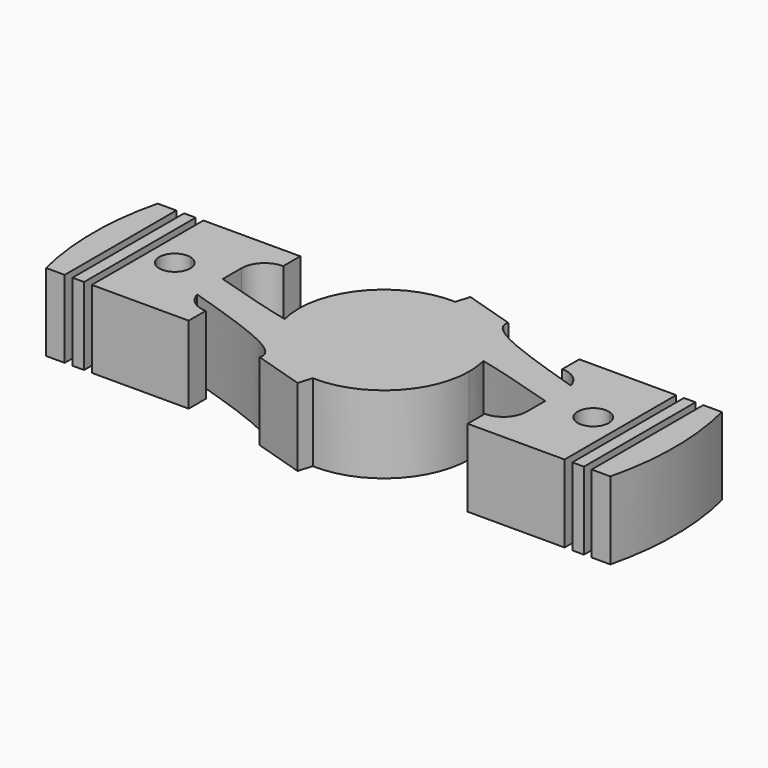
from build123d import *

# Parameters (mm, degrees)
F0_DEPTH = 25.4
F1_W     = 3.81
F1_H     = 45.72


with BuildPart() as f0:
    # F1 (on Top) → F0 (new body)
    with BuildSketch(Plane.XY):
        with BuildLine():
            Line((77.47, 22.86), (45.72, 22.86))
            Line((45.72, 22.86), (45.72, 15.875))
            ThreePointArc((45.72, 15.875), (50.3897919484, 14.2764153784), (53.1002511947, 10.1513892806))
            add(Edge.make_bspline(
                [(53.1002511947, 10.1513892806), (58.1589510072, 8.551724236), (63.812727866, 6.7977717351), (70.0851851843, 4.8518880408)],
                knots=[46.5844881463, 46.5844881463, 46.5844881463, 46.5844881463, 55.8862582945, 55.8862582945, 55.8862582945, 55.8862582945], degree=3))
            ThreePointArc((70.0851851843, 4.8518880408), (72.6697885481, 3.0133087515), (73.66, 0))
            ThreePointArc((73.66, 0), (71.5933087511, -4.0897885484), (67.0748148148, -4.8518880406))
            add(Edge.make_bspline(
                [(53.34, -0.6059576), (57.5451254916, -1.8955240295), (62.1166858374, -3.3137440808), (67.0748148148, -4.8518880406)],
                knots=[48.5335775556, 48.5335775556, 48.5335775556, 48.5335775556, 55.8862582953, 55.8862582953, 55.8862582953, 55.8862582953], degree=3))
            Line((53.34, -0.6059576), (53.34, -8.255))
            ThreePointArc((53.34, -8.255), (51.1081536726, -13.6431536726), (45.72, -15.875))
            Line((45.72, -15.875), (45.72, -22.86))
            Line((45.72, -22.86), (77.47, -22.86))
            Line((77.47, -22.86), (77.47, 22.86))
        make_face()
        with BuildLine():
            add(Edge.make_bspline(
                [(53.1002511947, 10.1513892806), (58.1589510072, 8.551724236), (63.812727866, 6.7977717351), (70.0851851843, 4.8518880408)],
                knots=[46.5844881463, 46.5844881463, 46.5844881463, 46.5844881463, 55.8862582945, 55.8862582945, 55.8862582945, 55.8862582945], degree=3))
            ThreePointArc((53.1002511947, 10.1513892806), (53.2798251998, 9.210742093), (53.34, 8.255))
            Line((53.34, 8.255), (53.34, -0.6059576))
            add(Edge.make_bspline(
                [(53.34, -0.6059576), (57.5451254916, -1.8955240295), (62.1166858374, -3.3137440808), (67.0748148148, -4.8518880406)],
                knots=[48.5335775556, 48.5335775556, 48.5335775556, 48.5335775556, 55.8862582953, 55.8862582953, 55.8862582953, 55.8862582953], degree=3))
            ThreePointArc((67.0748148148, -4.8518880406), (63.7281119593, 1.5051851848), (70.0851851843, 4.8518880408))
        make_face()
        with BuildLine():
            ThreePointArc((53.34, 8.255), (53.2798251998, 9.210742093), (53.1002511947, 10.1513892806))
            add(Edge.make_bspline(
                [(18.9075672089, 27.3046224959), (17.3563376005, 22.3043125946), (27.7656172811, 18.1627221903), (53.1002511947, 10.1513892806)],
                knots=[0, 0, 0, 0, 46.5844881463, 46.5844881463, 46.5844881463, 46.5844881463], degree=3))
            Line((18.9075672089, 27.3046224959), (2.4020174164, 32.4250846362))
            Line((2.4020174164, 32.4250846362), (1.0050151405, 27.9219187121))
            ThreePointArc((1.0050151405, 27.9219187121), (17.5750428532, 21.7200706423), (27.0976887869, 6.8087342735))
            add(Edge.make_bspline(
                [(27.0976887869, 6.8087342735), (33.4853412167, 5.3665593675), (42.104777648, 2.8394961928), (53.34, -0.6059576)],
                knots=[28.888740996, 28.888740996, 28.888740996, 28.888740996, 48.5335775556, 48.5335775556, 48.5335775556, 48.5335775556], degree=3))
            Line((53.34, -0.6059576), (53.34, 8.255))
        make_face()
        with BuildLine():
            ThreePointArc((27.94, 0), (27.7286226191, 3.4303188841), (27.0976887869, 6.8087342735))
            ThreePointArc((27.0976887869, 6.8087342735), (17.5750428532, 21.7200706423), (1.0050151405, 27.9219187121))
            ThreePointArc((1.0050151405, 27.9219187121), (-21.7200706423, 17.5750428532), (-27.0976887869, -6.8087342735))
            ThreePointArc((-27.0976887869, -6.8087342735), (-17.5750428532, -21.7200706423), (-1.0050151405, -27.9219187121))
            ThreePointArc((-1.0050151405, -27.9219187121), (19.3979828458, -20.108750869), (27.94, 0))
        make_face()
        with BuildLine():
            ThreePointArc((-1.0050151405, -27.9219187121), (-17.5750428532, -21.7200706423), (-27.0976887869, -6.8087342735))
            add(Edge.make_bspline(
                [(-27.0976887869, -6.8087342735), (-33.4853412167, -5.3665593675), (-42.104777648, -2.8394961928), (-53.34, 0.6059576)],
                knots=[28.888740996, 28.888740996, 28.888740996, 28.888740996, 48.5335775556, 48.5335775556, 48.5335775556, 48.5335775556], degree=3))
            Line((-53.34, 0.6059576), (-53.34, -8.255))
            ThreePointArc((-53.34, -8.255), (-53.2798251998, -9.210742093), (-53.1002511947, -10.1513892806))
            add(Edge.make_bspline(
                [(-18.9075672089, -27.3046224959), (-17.3563376005, -22.3043125946), (-27.7656172811, -18.1627221903), (-53.1002511947, -10.1513892806)],
                knots=[0, 0, 0, 0, 46.5844881463, 46.5844881463, 46.5844881463, 46.5844881463], degree=3))
            Line((-18.9075672089, -27.3046224959), (-2.4020174164, -32.4250846362))
            Line((-2.4020174164, -32.4250846362), (-1.0050151405, -27.9219187121))
        make_face()
        with BuildLine():
            add(Edge.make_bspline(
                [(-53.34, 0.6059576), (-57.5451254916, 1.8955240295), (-62.1166858374, 3.3137440808), (-67.0748148148, 4.8518880406)],
                knots=[48.5335775556, 48.5335775556, 48.5335775556, 48.5335775556, 55.8862582953, 55.8862582953, 55.8862582953, 55.8862582953], degree=3))
            Line((-53.34, 0.6059576), (-53.34, 8.255))
            ThreePointArc((-53.34, 8.255), (-51.1081536726, 13.6431536726), (-45.72, 15.875))
            Line((-45.72, 15.875), (-45.72, 22.86))
            Line((-45.72, 22.86), (-77.47, 22.86))
            Line((-77.47, 22.86), (-77.47, -22.86))
            Line((-77.47, -22.86), (-45.72, -22.86))
            Line((-45.72, -22.86), (-45.72, -15.875))
            ThreePointArc((-45.72, -15.875), (-50.3897919484, -14.2764153784), (-53.1002511947, -10.1513892806))
            add(Edge.make_bspline(
                [(-53.1002511947, -10.1513892806), (-58.1589510072, -8.551724236), (-63.812727866, -6.7977717351), (-70.0851851843, -4.8518880408)],
                knots=[46.5844881463, 46.5844881463, 46.5844881463, 46.5844881463, 55.8862582945, 55.8862582945, 55.8862582945, 55.8862582945], degree=3))
            ThreePointArc((-70.0851851843, -4.8518880408), (-73.4318880407, 1.5051851848), (-67.0748148148, 4.8518880406))
        make_face()
        with BuildLine():
            Line((-53.34, -8.255), (-53.34, 0.6059576))
            add(Edge.make_bspline(
                [(-53.34, 0.6059576), (-57.5451254916, 1.8955240295), (-62.1166858374, 3.3137440808), (-67.0748148148, 4.8518880406)],
                knots=[48.5335775556, 48.5335775556, 48.5335775556, 48.5335775556, 55.8862582953, 55.8862582953, 55.8862582953, 55.8862582953], degree=3))
            ThreePointArc((-67.0748148148, 4.8518880406), (-64.4902114516, 3.0133087511), (-63.5, 0))
            ThreePointArc((-63.5, 0), (-65.5666912485, -4.0897885481), (-70.0851851843, -4.8518880408))
            add(Edge.make_bspline(
                [(-53.1002511947, -10.1513892806), (-58.1589510072, -8.551724236), (-63.812727866, -6.7977717351), (-70.0851851843, -4.8518880408)],
                knots=[46.5844881463, 46.5844881463, 46.5844881463, 46.5844881463, 55.8862582945, 55.8862582945, 55.8862582945, 55.8862582945], degree=3))
            ThreePointArc((-53.1002511947, -10.1513892806), (-53.2798251998, -9.210742093), (-53.34, -8.255))
        make_face()
    extrude(amount=F0_DEPTH)


with BuildPart() as f0b:
    # F1 (on Top) → F0, piece 2 (new body)
    with BuildSketch(Plane.XY):
        with BuildLine():
            Line((92.4661175783, 22.86), (86.36, 22.86))
            Line((86.36, 22.86), (86.36, -22.86))
            Line((86.36, -22.86), (92.4661175783, -22.86))
            ThreePointArc((92.4661175783, -22.86), (95.25, 0), (92.4661175783, 22.86))
        make_face()
    extrude(amount=F0_DEPTH)


with BuildPart() as f0c:
    # F1 (on Top) → F0, piece 3 (new body)
    with BuildSketch(Plane.XY):
        with Locations((81.915, 0)):
            Rectangle(F1_W, F1_H)
    extrude(amount=F0_DEPTH)


with BuildPart() as f0d:
    # F1 (on Top) → F0, piece 4 (new body)
    with BuildSketch(Plane.XY):
        with Locations((-81.915, 0)):
            Rectangle(F1_W, F1_H)
    extrude(amount=F0_DEPTH)


with BuildPart() as f0e:
    # F1 (on Top) → F0, piece 5 (new body)
    with BuildSketch(Plane.XY):
        with BuildLine():
            Line((-92.4661175783, -22.86), (-86.36, -22.86))
            Line((-86.36, -22.86), (-86.36, 22.86))
            Line((-86.36, 22.86), (-92.4661175783, 22.86))
            ThreePointArc((-92.4661175783, 22.86), (-95.25, 0), (-92.4661175783, -22.86))
        make_face()
    extrude(amount=F0_DEPTH)


solid = Compound([f0.part, f0b.part, f0c.part, f0d.part, f0e.part])
